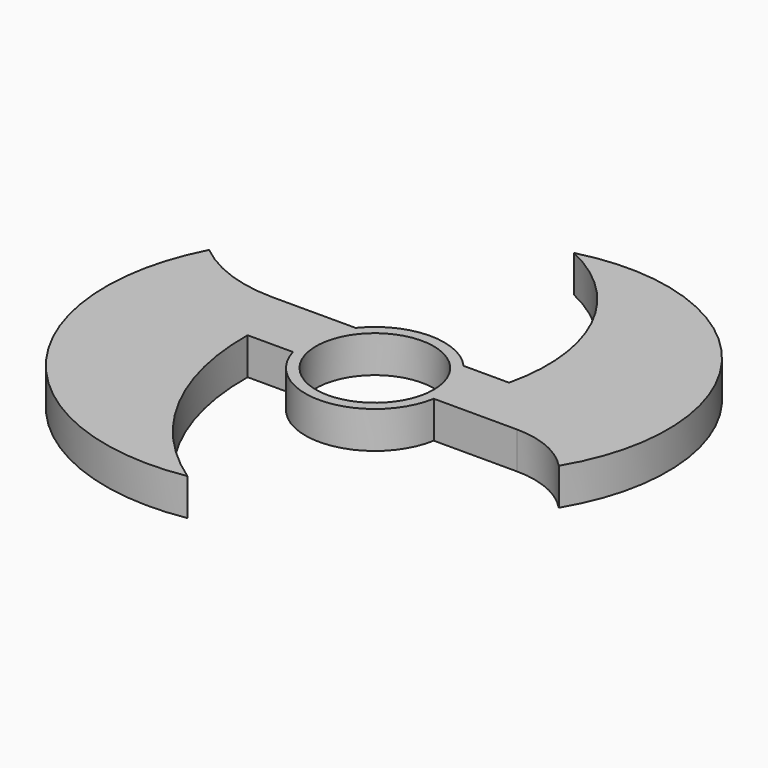
from build123d import *

# Parameters (mm, degrees)
F0_R     = 11.15
F1_DEPTH = 7


# Not quite as in the source:
# - a feature names something its author has since deleted; it is built from what else it names


with BuildPart() as f1:
    # F0 (on Top) → F1 (new body)
    with BuildSketch(Plane.XY):
        with BuildLine():
            ThreePointArc((-12.6572045799, -3.5661845468), (-12.883564121, 2.6336809867), (-10.2422641065, 8.2473344769))
            Line((-10.2422641065, 8.2473344769), (-26.0292641065, 8.2473344769))
            ThreePointArc((-26.0292641065, 8.2473344769), (-34.9143148349, 9.7844703454), (-42.7665638646, 14.217200689))
            ThreePointArc((-42.7665638646, 14.217200689), (-39.5806592619, -28.3580220296), (0, -44.3633645773))
            ThreePointArc((0, -44.3633645773), (-15.7763325785, -26.6479576979), (-21.2499108166, -3.5661845468))
            Line((-21.2499108166, -3.5661845468), (-12.6572045799, -3.5661845468))
        make_face()
        with BuildLine():
            ThreePointArc((12.9567624843, -2.2460645415), (13.1016015561, -1.1271808486), (13.15, 0))
            ThreePointArc((13.15, 0), (12.2942286487, 4.6663092411), (9.8382978048, 8.7252734229))
            ThreePointArc((9.8382978048, 8.7252734229), (-0.3128955133, 13.1462769025), (-10.2422641065, 8.2473344769))
            ThreePointArc((-10.2422641065, 8.2473344769), (-12.883564121, 2.6336809867), (-12.6572045799, -3.5661845468))
            ThreePointArc((-12.6572045799, -3.5661845468), (0.6768404107, -13.1325697051), (12.9567624843, -2.2460645415))
        make_face()
        Circle(F0_R, mode=Mode.SUBTRACT)
        with BuildLine():
            ThreePointArc((9.8382978048, 8.7252734229), (12.2942286487, 4.6663092411), (13.15, 0))
            ThreePointArc((13.15, 0), (13.1016015561, -1.1271808486), (12.9567624843, -2.2460645415))
            Line((12.9567624843, -2.2460645415), (28.7434491243, -2.2460645415))
            ThreePointArc((28.7434491243, -2.2460645415), (35.3157092291, -3.6070761232), (40.8069513167, -7.4662490586))
            ThreePointArc((40.8069513167, -7.4662490586), (38.839648653, 33.6212574976), (0, 47.1687726676))
            ThreePointArc((0, 47.1687726676), (16.0453137764, 31.2214280727), (18.4312978048, 8.7252734229))
            Line((18.4312978048, 8.7252734229), (9.8382978048, 8.7252734229))
        make_face()
    extrude(amount=F1_DEPTH)


solid = f1.part
